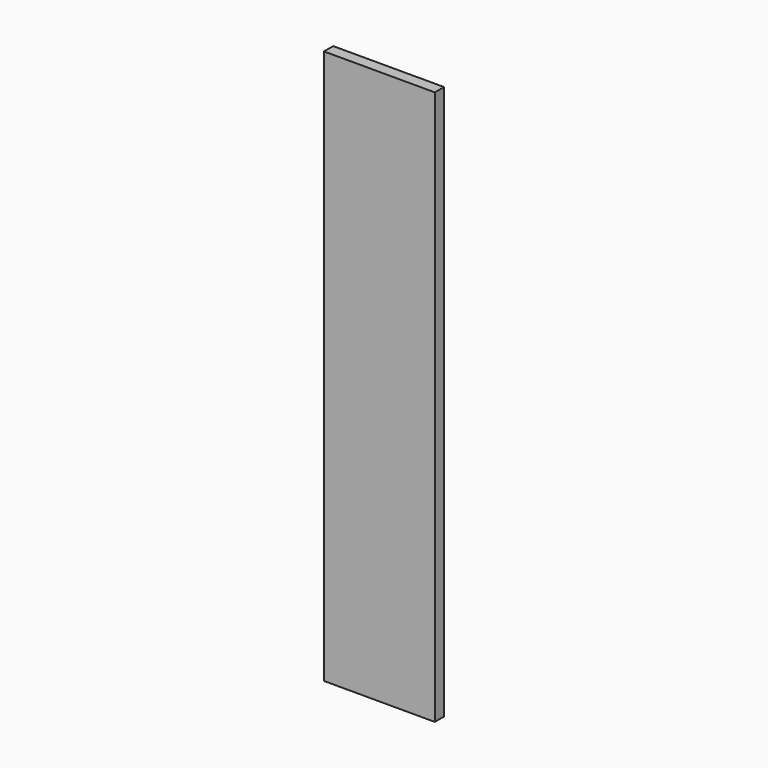
from build123d import *

# Parameters (mm, degrees)
F0_W     = 152.4
F0_H     = 762
F1_DEPTH = 15.875


# Not quite as in the source:
# - a length typed as a fraction of an inch, garbled in the dataset ("3 / 203.2 mm" for 3/8 in), is restored


with BuildPart() as f1:
    # F0 (on Front) → F1 (new body)
    with BuildSketch(Plane.XZ):
        with Locations((76.2, 381)):
            Rectangle(F0_W, F0_H)
    extrude(amount=F1_DEPTH)


solid = f1.part
